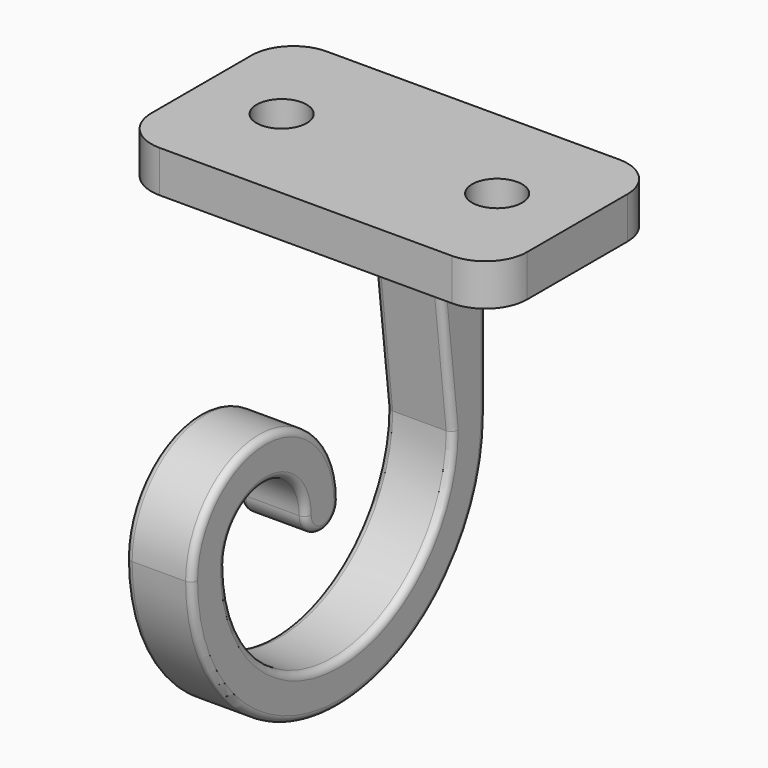
from build123d import *

# Parameters (mm, degrees)
F0_W     = 45
F0_H     = 25
F1_DEPTH = 5
F2_R     = 3
F3_DEPTH = 25
F6_DEPTH = 4
F7_W     = 8
F7_H     = 7.8920384722
F9_W     = 8
F9_H     = 5
F11_R    = 5
F12_R    = 0.8


# Not quite as in the source:
# - ends of sketch curves that miss each other by under 0.0002 mm in the source are joined


with BuildPart() as f1:
    # F0 (on Top) → F1 (new body)
    with BuildSketch(Plane.XY):
        with Locations((-11.3633279689, 6.0892301559)):
            Rectangle(F0_W, F0_H)
    extrude(amount=F1_DEPTH)

    # F2 (on face) → F3 (cut)
    with BuildSketch(Plane.XY.offset(5)):
        with Locations((-24.2633279689, 6.0892301559)):
            Circle(F2_R)
        with Locations((1.5366720311, 6.0892301559)):
            Circle(F2_R)
    extrude(amount=-F3_DEPTH, mode=Mode.SUBTRACT)

    # F5 (on line) → F6 (join, symmetric)
    with BuildSketch(Plane.YZ.offset(-11.3633279689)):
        with BuildLine():
            Line((15.5892301559, -25), (15.5892301559, 0))
            Line((15.5892301559, 0), (10.5892301559, 0))
            Line((10.5892301559, 0), (10.5892301559, -25))
            ThreePointArc((10.5892301559, -25), (-6.4107698441, -42), (-23.4107698441, -25))
            ThreePointArc((-23.4107698441, -25), (-17.4107695142, -19.0000002749), (-11.4107697891, -25))
            ThreePointArc((-11.4107697891, -25), (-8.9107696516, -27.5), (-6.4107696516, -25))
            ThreePointArc((-6.4107696516, -25), (-17.4107695142, -14), (-28.4107695142, -25))
            ThreePointArc((-28.4107695142, -25), (-6.4107698441, -47), (15.5892301559, -25))
        make_face()
    extrude(amount=F6_DEPTH, both=True)

    # F7 (on face) → F10 section 0
    with BuildSketch(Plane.XY):
        with Locations((-11.3633279689, 11.6432109198)):
            Rectangle(F7_W, F7_H)
    # F9 (on face) → F10 section 1
    with BuildSketch(Plane.XY.offset(-25)):
        with Locations((-11.3633279689, 13.0892301559)):
            Rectangle(F9_W, F9_H)
    loft()

    # F11
    f11_edges = [f1.edges().sort_by_distance(p)[0] for p in [
        (-33.863328, 18.58923, 2.5),
        (-33.863328, -6.41077, 2.5),
        (11.136672, 18.58923, 2.5),
        (11.136672, -6.41077, 2.5),
    ]]
    fillet(f11_edges, radius=F11_R)

    # F12
    f12_edges = [f1.edges().sort_by_distance(p)[0] for p in [
        (-7.363328, 15.58923, -12.5),
        (-7.363328, -6.41077, -47),
        (-15.363328, 15.58923, -12.5),
        (-15.363328, -6.41077, -47),
        (-15.363328, 9.143211, -12.5),
        (-7.363328, 9.143211, -12.5),
    ]]
    fillet(f12_edges, radius=F12_R)


solid = f1.part
